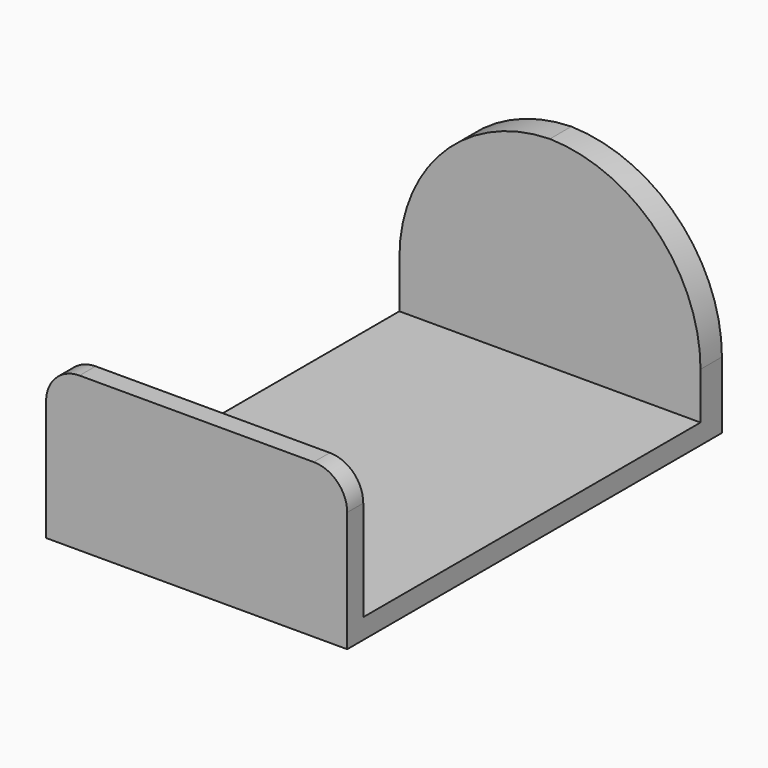
from build123d import *

# Parameters (mm, degrees)
F0_W        = 45
F0_H        = 70
F1_DEPTH    = 3
F2_W        = 45
F2_H        = 4
F3_DEPTH    = 30
F4_T1_DEPTH = 119
F5_W        = 45
F5_H        = 3
F6_DEPTH    = 20
F7_R        = 5


# Not quite as in the source:
# - a fillet or chamfer that OpenCascade refuses, or shapes differently, is made with other operations: its cross-section is extruded or revolved along the edge and cut away or added


with BuildPart() as f1:
    # F0 (on Top) → F1 (new body)
    with BuildSketch(Plane.XY):
        Rectangle(F0_W, F0_H)
    extrude(amount=F1_DEPTH)

    # F2 (on face) → F3 (join)
    with BuildSketch(Plane.XY.offset(3)):
        with Locations((0, 33)):
            Rectangle(F2_W, F2_H)
    extrude(amount=F3_DEPTH)

    # F4: fillet of radius 23 on 2 edges, made by hand

    # F4_s2 → F4_t1 (cut)
    with BuildSketch(Plane.XZ.offset(-92.5)):
        with BuildLine():
            ThreePointArc((-22.5, 10), (-15.7634559673, 26.2634559673), (0.5, 33))
            Line((0.5, 33), (-22.5, 33))
            Line((-22.5, 33), (-22.5, 10))
        make_face()
        with BuildLine():
            ThreePointArc((-0.5, 33), (15.7634559673, 26.2634559673), (22.5, 10))
            Line((22.5, 10), (22.5, 33))
            Line((22.5, 33), (-0.5, 33))
        make_face()
    extrude(amount=F4_T1_DEPTH, mode=Mode.SUBTRACT)

    # F5 (on face) → F6 (join)
    with BuildSketch(Plane.XY.offset(3)):
        with Locations((0, -33.5)):
            Rectangle(F5_W, F5_H)
    extrude(amount=F6_DEPTH)

    # F7
    f7_edges = [f1.edges().sort_by_distance(p)[0] for p in [
        (-22.5, -33.5, 23),
        (22.5, -33.5, 23),
    ]]
    fillet(f7_edges, radius=F7_R)


solid = f1.part
